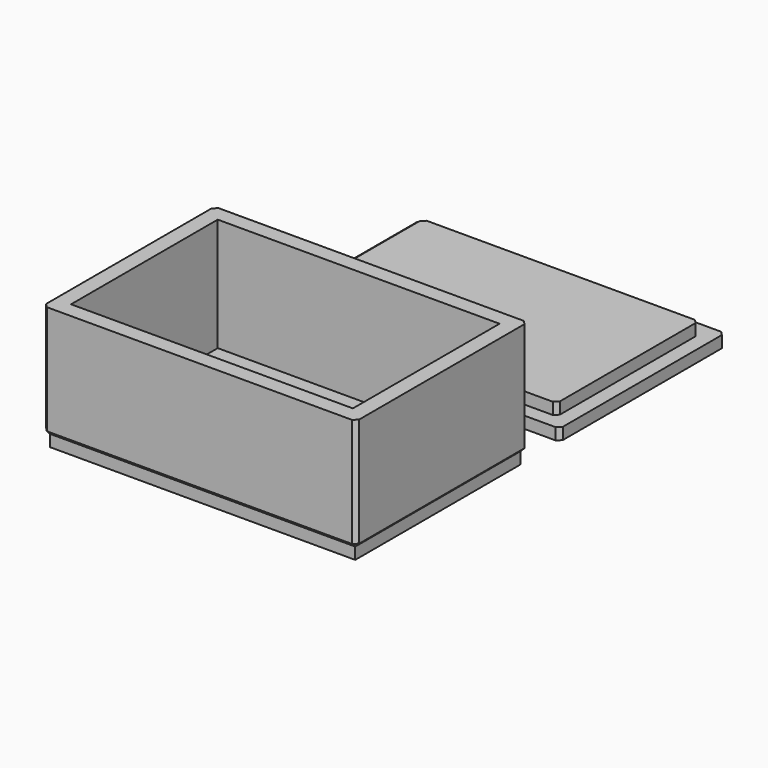
from build123d import *

# Parameters (mm, degrees)
F0_W      = 31.3
F0_H      = 21.2
F1_DEPTH  = 1.2
F2_W      = 32.1
F2_H      = 22
F2_W_2    = 31.3
F2_H_2    = 21.2
F2_W_3    = 28.9
F2_H_3    = 18.8
F3_DEPTH  = 11.6
F4_W      = 28.3
F4_H      = 18.2
F5_DEPTH  = 1.2
F6_SIZE   = 0.39999
F6_2_SIZE = 0.39999


# Not quite as in the source:
# - a fillet or chamfer is up to 0.001 mm smaller than in the source, because OpenCascade refuses the exact size


with BuildPart() as f1:
    # F0 (on Top) → F1 (new body)
    with BuildSketch(Plane.XY):
        Rectangle(F0_W, F0_H)
    extrude(amount=F1_DEPTH)

    # F2 (on face) → F3 (join)
    with BuildSketch(Plane.XY.offset(1.2)):
        Rectangle(F2_W, F2_H)
        Rectangle(F2_W_2, F2_H_2, mode=Mode.SUBTRACT)
        Rectangle(F2_W_2, F2_H_2)
        Rectangle(F2_W_3, F2_H_3, mode=Mode.SUBTRACT)
    extrude(amount=F3_DEPTH)

    # F6 (size 0.4 in the source; OpenCascade refuses exactly that, so slightly less here)
    f6_edges = [f1.edges().sort_by_distance(p)[0] for p in [
        (-16.05, 0, 1.2),
        (0, -11, 1.2),
        (16.05, 0, 1.2),
        (0, 11, 1.2),
        (-16.05, -11, 7),
        (16.05, -11, 7),
        (16.05, 11, 7),
        (-16.05, 11, 7),
    ]]
    chamfer(f6_edges, length=F6_SIZE)


with BuildPart() as f1b:
    # F0 (on Top) → F1, piece 2 (new body)
    with BuildSketch(Plane.XY):
        with Locations((0, 26.2)):
            Rectangle(F0_W, F0_H)
    extrude(amount=F1_DEPTH)

    # F4 (on face) → F5 (join)
    with BuildSketch(Plane.XY.offset(1.2)):
        with Locations((0, 26.2)):
            Rectangle(F4_W, F4_H)
    extrude(amount=F5_DEPTH)

    # F6#2 (size 0.4 in the source; OpenCascade refuses exactly that, so slightly less here)
    f6_2_edges = [f1b.edges().sort_by_distance(p)[0] for p in [
        (15.65, 36.8, 0.6),
        (15.65, 15.6, 0.6),
        (-15.65, 36.8, 0.6),
        (-14.15, 35.3, 1.8),
        (14.15, 35.3, 1.8),
        (14.15, 17.1, 1.8),
        (-14.15, 17.1, 1.8),
        (-15.65, 15.6, 0.6),
    ]]
    chamfer(f6_2_edges, length=F6_2_SIZE)


solid = Compound([f1.part, f1b.part])
